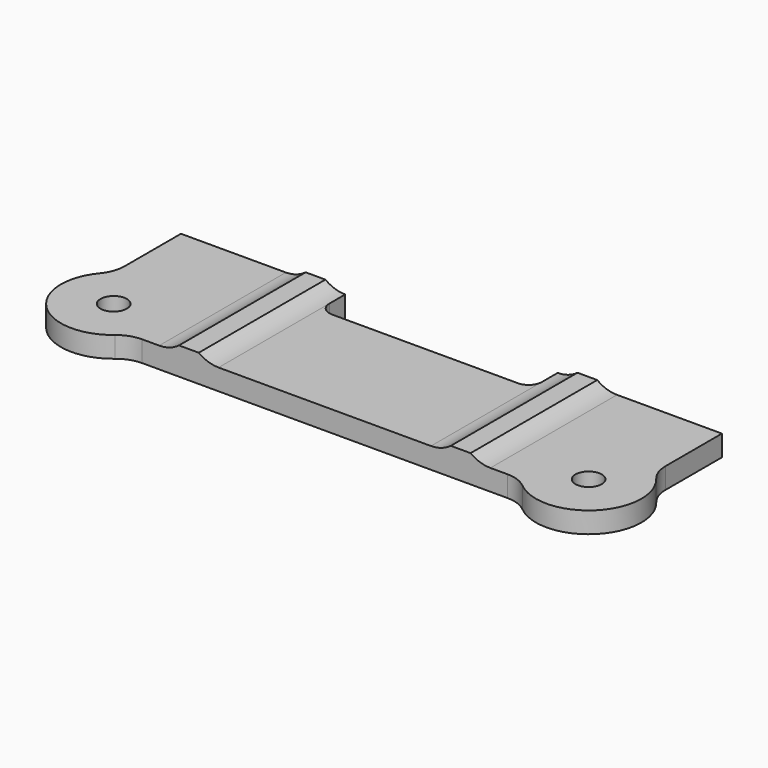
from build123d import *

# Parameters (mm, degrees)
F0_R        = 2
F1_DEPTH    = 3.175
F2_R        = 5
F3_R        = 2
F4_W        = 3
F4_H        = 24
F5_DEPTH    = 1
F6_T1_DEPTH = 24


# Not quite as in the source:
# - a fillet or chamfer that OpenCascade refuses, or shapes differently, is made with other operations: its cross-section is extruded or revolved along the edge and cut away or added


with BuildPart() as f1:
    # F0 (on Top) → F1 (new body)
    with BuildSketch(Plane.XY):
        with BuildLine():
            Line((11.2449979984, 0), (0, 0))
            Line((0, 0), (0, 11.2449979984))
            ThreePointArc((0, 11.2449979984), (-0.6568542495, -0.6568542495), (11.2449979984, 0))
        make_face()
        Polygon((0, 11.2449979984), (0, 0), (11.2449979984, 0), (41, 0), (70.7550020016, 0), (82, 0), (82, 11.2449979984), (82, 24), (57.1, 24), (57.1, 19), (41, 19), (24.9, 19), (24.9, 24), (0, 24), align=None)
        with Locations((5, 5)):
            Circle(F0_R, mode=Mode.SUBTRACT)
        with Locations((77, 5)):
            Circle(F0_R, mode=Mode.SUBTRACT)
        with BuildLine():
            Line((82, 0), (70.7550020016, 0))
            ThreePointArc((70.7550020016, 0), (82.6568542495, -0.6568542495), (82, 11.2449979984))
            Line((82, 11.2449979984), (82, 0))
        make_face()
    extrude(amount=F1_DEPTH)

    # F2
    f2_edges = [f1.edges().sort_by_distance(p)[0] for p in [
        (11.244998, 0, 1.5875),
        (70.755002, 0, 1.5875),
        (82, 11.244998, 1.5875),
        (0, 11.244998, 1.5875),
    ]]
    fillet(f2_edges, radius=F2_R)

    # F3
    f3_edges = [f1.edges().sort_by_distance(p)[0] for p in [
        (24.9, 19, 1.5875),
        (57.1, 19, 1.5875),
    ]]
    fillet(f3_edges, radius=F3_R)

    # F4 (on face) → F5 (join)
    with BuildSketch(Plane.XY.offset(3.175)):
        with Locations((20.4, 12)):
            Rectangle(F4_W, F4_H)
        with Locations((61.6, 12)):
            Rectangle(F4_W, F4_H)
    extrude(amount=F5_DEPTH)

    # F6: fillet of radius 5 on 4 edges, made by hand

    # F6_s2 → F6_t1 (join)
    with BuildSketch(Plane.XZ.offset(-24)):
        with BuildLine():
            ThreePointArc((15.9, 3.175), (17.4811388301, 3.4315835097), (18.9, 4.175))
            Line((18.9, 4.175), (18.96, 4.095))
            ThreePointArc((18.96, 4.095), (19, 3.675), (19, 3.175))
            Line((19, 3.175), (18.9, 3.075))
            Line((18.9, 3.075), (15.9, 3.075))
            Line((15.9, 3.075), (15.9, 3.175))
        make_face()
        with BuildLine():
            ThreePointArc((24.9, 3.175), (23.3188611699, 3.4315835097), (21.9, 4.175))
            Line((21.9, 4.175), (21.84, 4.095))
            ThreePointArc((21.84, 4.095), (21.8, 3.675), (21.8, 3.175))
            Line((21.8, 3.175), (21.9, 3.075))
            Line((21.9, 3.075), (24.9, 3.075))
            Line((24.9, 3.075), (24.9, 3.175))
        make_face()
        with BuildLine():
            ThreePointArc((57.1, 3.175), (58.6811388301, 3.4315835097), (60.1, 4.175))
            Line((60.1, 4.175), (60.16, 4.095))
            ThreePointArc((60.16, 4.095), (60.2, 3.675), (60.2, 3.175))
            Line((60.2, 3.175), (60.1, 3.075))
            Line((60.1, 3.075), (57.1, 3.075))
            Line((57.1, 3.075), (57.1, 3.175))
        make_face()
        with BuildLine():
            ThreePointArc((66.1, 3.175), (64.5188611699, 3.4315835097), (63.1, 4.175))
            Line((63.1, 4.175), (63.04, 4.095))
            ThreePointArc((63.04, 4.095), (63, 3.675), (63, 3.175))
            Line((63, 3.175), (63.1, 3.075))
            Line((63.1, 3.075), (66.1, 3.075))
            Line((66.1, 3.075), (66.1, 3.175))
        make_face()
    extrude(amount=F6_T1_DEPTH)


solid = f1.part
